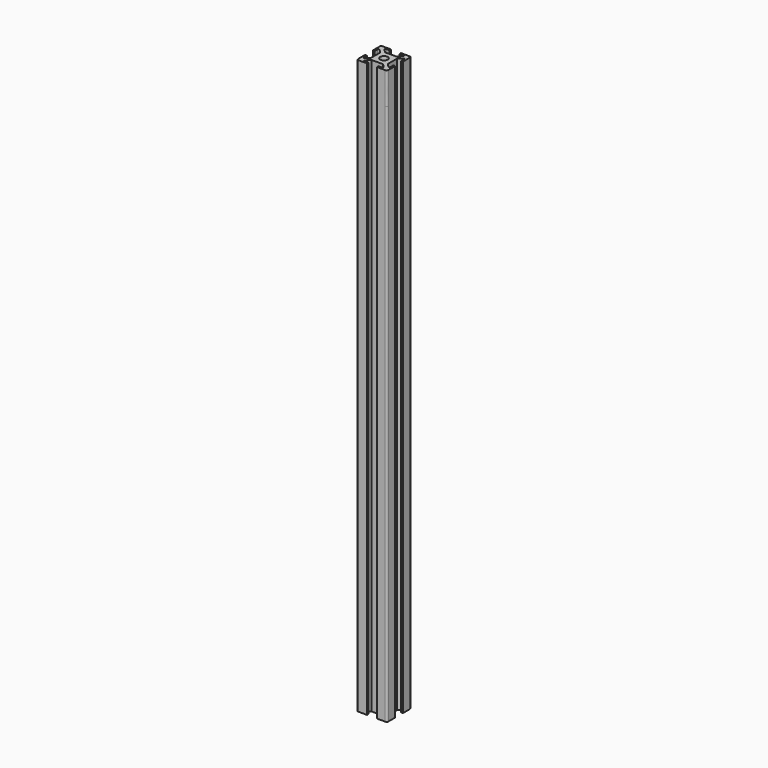
from build123d import *

# Parameters (mm, degrees)
F0_W        = 25.4
F0_H        = 25.4
F1_DEPTH    = 455.93
F3_DEPTH    = 455.93
F4_R        = 3.175
F5_DEPTH    = 455.93
F6_T1_DEPTH = 463.8675
F7_T1_DEPTH = 455.93
F8_DEPTH    = 26.67


# Not quite as in the source:
# - a fillet or chamfer that OpenCascade refuses, or shapes differently, is made with other operations: its cross-section is extruded or revolved along the edge and cut away or added


with BuildPart() as f1:
    # F0 (on Top) → F1 (new body)
    with BuildSketch(Plane.XY):
        Rectangle(F0_W, F0_H)
    extrude(amount=F1_DEPTH)

    # F2 (on face) → F3 (cut)
    with BuildSketch(Plane.XY.offset(455.93)):
        Polygon((-7.0075640303, -4.7625), (-7.0075640303, 4.7625), (-11.1125, 8.8674359697), (-11.1125, 4.1049359697), (-12.7, 4.1049359697), (-12.7, -4.1049359697), (-11.1125, -4.1049359697), (-11.1125, -8.8674359697), align=None)
        Polygon((4.1049359697, 12.7), (-4.1049359697, 12.7), (-4.1049359697, 11.1125), (-8.8674359697, 11.1125), (-4.7625, 7.0075640303), (4.7625, 7.0075640303), (8.8674359697, 11.1125), (4.1049359697, 11.1125), align=None)
        Polygon((12.7, -4.1049359697), (12.7, 4.1049359697), (11.1125, 4.1049359697), (11.1125, 8.8674359697), (7.0075640303, 4.7625), (7.0075640303, -4.7625), (11.1125, -8.8674359697), (11.1125, -4.1049359697), align=None)
        Polygon((-4.1049359697, -11.1125), (-4.1049359697, -12.7), (4.1049359697, -12.7), (4.1049359697, -11.1125), (8.8674359697, -11.1125), (4.7625, -7.0075640303), (-4.7625, -7.0075640303), (-8.8674359697, -11.1125), align=None)
    extrude(amount=-F3_DEPTH, mode=Mode.SUBTRACT)

    # F4 (on face) → F5 (cut)
    with BuildSketch(Plane.XY.offset(455.93)):
        Circle(F4_R)
    extrude(amount=-F5_DEPTH, mode=Mode.SUBTRACT)

    # F6: fillet of radius 1.5875 on 4 edges, made by hand

    # F6_s2 → F6_t1 (cut)
    with BuildSketch(Plane.XY.offset(-3.96875)):
        with BuildLine():
            add(Edge.make_bspline(
                [(-12.7, 11.1125), (-12.7, 12.7), (-11.1125, 12.7)],
                knots=[0, 0, 0, 1, 1, 1], degree=2, weights=[1, 1, 1]))
            Line((-11.1125, 12.7), (-12.7, 12.7))
            Line((-12.7, 12.7), (-12.7, 11.1125))
        make_face()
        with BuildLine():
            add(Edge.make_bspline(
                [(12.7, 11.1125), (12.7, 12.7), (11.1125, 12.7)],
                knots=[0, 0, 0, 1, 1, 1], degree=2, weights=[1, 1, 1]))
            Line((11.1125, 12.7), (12.7, 12.7))
            Line((12.7, 12.7), (12.7, 11.1125))
        make_face()
        with BuildLine():
            add(Edge.make_bspline(
                [(12.7, -11.1125), (12.7, -12.7), (11.1125, -12.7)],
                knots=[0, 0, 0, 1, 1, 1], degree=2, weights=[1, 1, 1]))
            Line((11.1125, -12.7), (12.7, -12.7))
            Line((12.7, -12.7), (12.7, -11.1125))
        make_face()
        with BuildLine():
            add(Edge.make_bspline(
                [(-11.1125, -12.7), (-12.7, -12.7), (-12.7, -11.1125)],
                knots=[0, 0, 0, 1, 1, 1], degree=2, weights=[1, 1, 1]))
            Line((-12.7, -11.1125), (-12.7, -12.7))
            Line((-12.7, -12.7), (-11.1125, -12.7))
        make_face()
    extrude(amount=F6_T1_DEPTH, mode=Mode.SUBTRACT)

    # F7: fillet of radius 0.79375 on 8 edges, made by hand

    # F7_s2 → F7_t1 (join)
    with BuildSketch(Plane.XY):
        with BuildLine():
            add(Edge.make_bspline(
                [(-9.7574839924, 7.5124199622), (-11.1125, 8.8674359697), (-11.1125, 6.9511539546)],
                knots=[0, 0, 0, 1, 1, 1], degree=2, weights=[1, 1, 1]))
            Line((-11.1125, 6.9511539546), (-11.1125, 8.8674359697))
            Line((-11.1125, 8.8674359697), (-9.7574839924, 7.5124199622))
        make_face()
        with BuildLine():
            add(Edge.make_bspline(
                [(11.1125, 6.9511539546), (11.1125, 8.8674359697), (9.7574839924, 7.5124199622)],
                knots=[0, 0, 0, 1, 1, 1], degree=2, weights=[1, 1, 1]))
            Line((9.7574839924, 7.5124199622), (11.1125, 8.8674359697))
            Line((11.1125, 8.8674359697), (11.1125, 6.9511539546))
        make_face()
        with BuildLine():
            add(Edge.make_bspline(
                [(9.7574839924, -7.5124199622), (11.1125, -8.8674359697), (11.1125, -6.9511539546)],
                knots=[0, 0, 0, 1, 1, 1], degree=2, weights=[1, 1, 1]))
            Line((11.1125, -6.9511539546), (11.1125, -8.8674359697))
            Line((11.1125, -8.8674359697), (9.7574839924, -7.5124199622))
        make_face()
        with BuildLine():
            add(Edge.make_bspline(
                [(-11.1125, -6.9511539546), (-11.1125, -8.8674359697), (-9.7574839924, -7.5124199622)],
                knots=[0, 0, 0, 1, 1, 1], degree=2, weights=[1, 1, 1]))
            Line((-9.7574839924, -7.5124199622), (-11.1125, -8.8674359697))
            Line((-11.1125, -8.8674359697), (-11.1125, -6.9511539546))
        make_face()
        with BuildLine():
            add(Edge.make_bspline(
                [(-7.5124199622, -9.7574839924), (-8.8674359697, -11.1125), (-6.9511539546, -11.1125)],
                knots=[0, 0, 0, 1, 1, 1], degree=2, weights=[1, 1, 1]))
            Line((-6.9511539546, -11.1125), (-8.8674359697, -11.1125))
            Line((-8.8674359697, -11.1125), (-7.5124199622, -9.7574839924))
        make_face()
        with BuildLine():
            add(Edge.make_bspline(
                [(6.9511539546, -11.1125), (8.8674359697, -11.1125), (7.5124199622, -9.7574839924)],
                knots=[0, 0, 0, 1, 1, 1], degree=2, weights=[1, 1, 1]))
            Line((7.5124199622, -9.7574839924), (8.8674359697, -11.1125))
            Line((8.8674359697, -11.1125), (6.9511539546, -11.1125))
        make_face()
        with BuildLine():
            add(Edge.make_bspline(
                [(7.5124199622, 9.7574839924), (8.8674359697, 11.1125), (6.9511539546, 11.1125)],
                knots=[0, 0, 0, 1, 1, 1], degree=2, weights=[1, 1, 1]))
            Line((6.9511539546, 11.1125), (8.8674359697, 11.1125))
            Line((8.8674359697, 11.1125), (7.5124199622, 9.7574839924))
        make_face()
        with BuildLine():
            add(Edge.make_bspline(
                [(-6.9511539546, 11.1125), (-8.8674359697, 11.1125), (-7.5124199622, 9.7574839924)],
                knots=[0, 0, 0, 1, 1, 1], degree=2, weights=[1, 1, 1]))
            Line((-7.5124199622, 9.7574839924), (-8.8674359697, 11.1125))
            Line((-8.8674359697, 11.1125), (-6.9511539546, 11.1125))
        make_face()
    extrude(amount=F7_T1_DEPTH)

    # F8 (add): a face of the model
    f8_faces = [f1.faces().sort_by_distance(p)[0] for p in [
        (4.4641462174, -11.90625, 455.93),
    ]]
    extrude(f8_faces, amount=F8_DEPTH)


solid = f1.part
